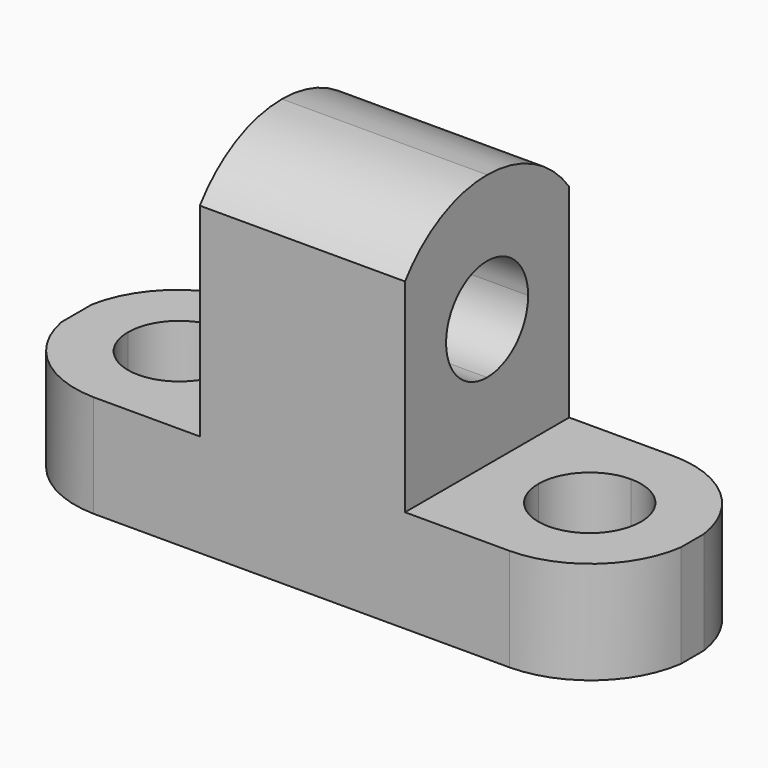
from build123d import *

# Parameters (mm, degrees)
F0_W     = 76.2
F0_H     = 44.45
F1_DEPTH = 25.4
F2_W     = 25.4
F2_H     = 31.75
F3_DEPTH = 25.4
F5_DEPTH = 25.4
F7_DEPTH = 25.4
F9_DEPTH = 25.4


with BuildPart() as f1:
    # F0 (on Front) → F1 (new body)
    with BuildSketch(Plane.XZ):
        with Locations((38.1, 22.225)):
            Rectangle(F0_W, F0_H)
    extrude(amount=F1_DEPTH)

    # F2 (on face) → F3 (cut)
    with BuildSketch(Plane.XZ.offset(25.4)):
        with Locations((12.7, 28.575)):
            Rectangle(F2_W, F2_H)
        with Locations((63.5, 28.575)):
            Rectangle(F2_W, F2_H)
    extrude(amount=-F3_DEPTH, mode=Mode.SUBTRACT)

    # F4 (on face) → F5 (cut)
    with BuildSketch(Plane.YZ.offset(50.8)):
        with BuildLine():
            Line((-12.7, 28.575), (-12.7, 34.925))
            ThreePointArc((-12.7, 34.925), (-17.1901280605, 33.0651280605), (-19.05, 28.575))
            Line((-19.05, 28.575), (-12.7, 28.575))
        make_face()
        with BuildLine():
            ThreePointArc((-6.35, 28.575), (-8.2098719395, 33.0651280605), (-12.7, 34.925))
            Line((-12.7, 34.925), (-12.7, 28.575))
            Line((-12.7, 28.575), (-6.35, 28.575))
        make_face()
        with BuildLine():
            Line((-6.35, 28.575), (-12.7, 28.575))
            Line((-12.7, 28.575), (-12.7, 22.225))
            ThreePointArc((-12.7, 22.225), (-8.2098719395, 24.0848719395), (-6.35, 28.575))
        make_face()
        with BuildLine():
            Line((-12.7, 22.225), (-12.7, 28.575))
            Line((-12.7, 28.575), (-19.05, 28.575))
            ThreePointArc((-19.05, 28.575), (-17.1901280605, 24.0848719395), (-12.7, 22.225))
        make_face()
        with BuildLine():
            Line((-12.7, 44.3012688375), (-12.7, 44.45))
            Line((-12.7, 44.45), (-25.4, 44.45))
            Line((-25.4, 44.45), (-25.4, 37.8499949622))
            ThreePointArc((-25.4, 37.8499949622), (-19.8223053609, 42.5959948968), (-12.7, 44.3012688375))
        make_face()
        with BuildLine():
            Line((0, 44.45), (-12.7, 44.45))
            Line((-12.7, 44.45), (-12.7, 44.3012688375))
            ThreePointArc((-12.7, 44.3012688375), (-5.5776946391, 42.5959948968), (0, 37.8499949622))
            Line((0, 37.8499949622), (0, 44.45))
        make_face()
    extrude(amount=-F5_DEPTH, mode=Mode.SUBTRACT)

    # F6 (on face) → F7 (cut)
    with BuildSketch(Plane.XY.offset(12.7)):
        with BuildLine():
            Line((6.35, -12.7), (12.7, -12.7))
            Line((12.7, -12.7), (12.7, -6.35))
            ThreePointArc((12.7, -6.35), (8.2098719395, -8.2098719395), (6.35, -12.7))
        make_face()
        with BuildLine():
            Line((12.7, -12.7), (19.05, -12.7))
            ThreePointArc((19.05, -12.7), (17.1901280605, -8.2098719395), (12.7, -6.35))
            Line((12.7, -6.35), (12.7, -12.7))
        make_face()
        with BuildLine():
            Line((12.7, -19.05), (12.7, -12.7))
            Line((12.7, -12.7), (6.35, -12.7))
            ThreePointArc((6.35, -12.7), (8.2098719395, -17.1901280605), (12.7, -19.05))
        make_face()
        with BuildLine():
            ThreePointArc((12.7, -19.05), (17.1901280605, -17.1901280605), (19.05, -12.7))
            Line((19.05, -12.7), (12.7, -12.7))
            Line((12.7, -12.7), (12.7, -19.05))
        make_face()
        with BuildLine():
            ThreePointArc((0, -10.327417444), (4.2938587705, -2.9864667778), (12.2567600012, 0))
            Line((12.2567600012, 0), (0, 0))
            Line((0, 0), (0, -10.327417444))
        make_face()
        with BuildLine():
            Line((0, -25.4), (12.2567600012, -25.4))
            ThreePointArc((12.2567600012, -25.4), (4.2938587705, -22.4135332222), (0, -15.072582556))
            Line((0, -15.072582556), (0, -25.4))
        make_face()
    extrude(amount=-F7_DEPTH, mode=Mode.SUBTRACT)

    # F8 (on face) → F9 (cut)
    with BuildSketch(Plane.XY.offset(12.7)):
        with BuildLine():
            ThreePointArc((63.5, -19.05), (67.9901280605, -17.1901280605), (69.85, -12.7))
            Line((69.85, -12.7), (63.5, -12.7))
            Line((63.5, -12.7), (63.5, -19.05))
        make_face()
        with BuildLine():
            Line((63.5, -12.7), (69.85, -12.7))
            ThreePointArc((69.85, -12.7), (67.9901280605, -8.2098719395), (63.5, -6.35))
            Line((63.5, -6.35), (63.5, -12.7))
        make_face()
        with BuildLine():
            Line((63.5, -19.05), (63.5, -12.7))
            Line((63.5, -12.7), (57.15, -12.7))
            ThreePointArc((57.15, -12.7), (59.0098719395, -17.1901280605), (63.5, -19.05))
        make_face()
        with BuildLine():
            Line((57.15, -12.7), (63.5, -12.7))
            Line((63.5, -12.7), (63.5, -6.35))
            ThreePointArc((63.5, -6.35), (59.0098719395, -8.2098719395), (57.15, -12.7))
        make_face()
        with BuildLine():
            Line((76.2, -25.4), (76.2, -14.4800225697))
            ThreePointArc((76.2, -14.4800225697), (71.9993464021, -22.2483812307), (63.7494866416, -25.4))
            Line((63.7494866416, -25.4), (76.2, -25.4))
        make_face()
        with BuildLine():
            ThreePointArc((63.7494866416, 0), (71.9993464021, -3.1516187693), (76.2, -10.9199774303))
            Line((76.2, -10.9199774303), (76.2, 0))
            Line((76.2, 0), (63.7494866416, 0))
        make_face()
    extrude(amount=-F9_DEPTH, mode=Mode.SUBTRACT)


solid = f1.part
